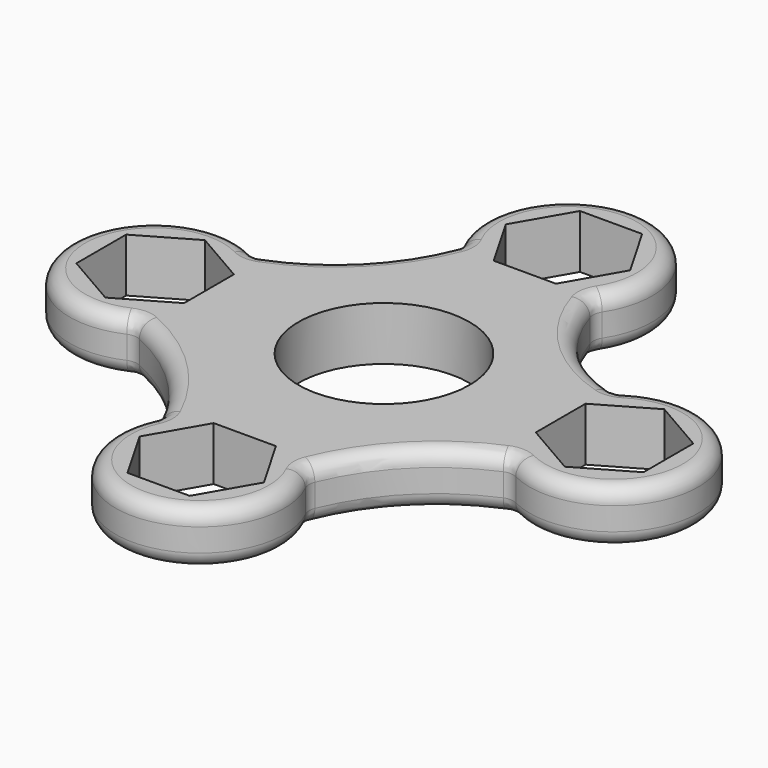
from build123d import *

# Parameters (mm, degrees)
F0_R     = 11.15
F1_DEPTH = 7
F2_F1_R  = 2
F2_F2_R  = 2


with BuildPart() as f1:
    # F0 (on Top) → F1 (new body)
    with BuildSketch(Plane.XY):
        with BuildLine():
            ThreePointArc((23.3964503772, 8.797336664), (14.0846149988, 14.053375372), (8.7316436817, 23.3098282073))
            ThreePointArc((8.7316436817, 23.3098282073), (0.5437011827, 40.9865549206), (-9.3495266884, 24.2046267848))
            ThreePointArc((-9.3495266884, 24.2046267848), (-15.072406885, 15.069278283), (-24.2129318757, 9.3546695572))
            ThreePointArc((-24.2129318757, 9.3546695572), (-40.995618633, 0.310436593), (-24.7499456016, -9.6662779194))
            ThreePointArc((-24.7499456016, -9.6662779194), (-15.7123412284, -15.6876267313), (-9.6305294082, -24.6846539794))
            ThreePointArc((-9.6305294082, -24.6846539794), (0.1339060787, -40.9991849317), (9.4982743355, -24.4517764422))
            ThreePointArc((9.4982743355, -24.4517764422), (15.2376463276, -15.298425789), (24.29093254, -9.4024756707))
            ThreePointArc((24.29093254, -9.4024756707), (40.9867386931, 0.5399748969), (23.3964503772, 8.797336664))
        make_face()
        Polygon((-3.9538544588, -36.8794909641), (-8.0114721507, -29.8514909641), (-3.9538544588, -22.8234909641), (4.1613809249, -22.8234909641), (8.2189986168, -29.8514909641), (4.1613809249, -36.8794909641), align=None, mode=Mode.SUBTRACT)
        Polygon((-36.9018638655, 4.0799905933), (-29.8738638655, 8.1376082852), (-22.8458638655, 4.0799905933), (-22.8458638655, -4.0352447904), (-29.8738638655, -8.0928624823), (-36.9018638655, -4.0352447904), align=None, mode=Mode.SUBTRACT)
        Circle(F0_R, mode=Mode.SUBTRACT)
        Polygon((8.1152353837, 30), (4.0576176919, 22.972), (-4.0576176919, 22.972), (-8.1152353837, 30), (-4.0576176919, 37.028), (4.0576176919, 37.028), align=None, mode=Mode.SUBTRACT)
        Polygon((37.0056270986, -3.9314815574), (29.9776270986, -7.9890992492), (22.9496270986, -3.9314815574), (22.9496270986, 4.1837538264), (29.9776270986, 8.2413715182), (37.0056270986, 4.1837538264), align=None, mode=Mode.SUBTRACT)
    extrude(amount=F1_DEPTH)

    # F2: fillet of radius 2 on 16 edges, made by hand

    # F2_f1
    f2_f1_edges = [f1.edges().sort_by_distance(p)[0] for p in [
        (-24.2129318757, 9.3546695572, 3.5),
        (-24.7499456016, -9.6662779194, 3.5),
        (-9.6305294082, -24.6846539794, 3.5),
        (9.4982743355, -24.4517764422, 3.5),
        (24.29093254, -9.4024756707, 3.5),
        (23.3964503772, 8.797336664, 3.5),
        (8.7316436817, 23.3098282073, 3.5),
        (-9.3495266884, 24.2046267848, 3.5),
    ]]
    fillet(f2_f1_edges, radius=F2_F1_R)

    # F2_f2
    f2_f2_edges = [f1.edges().sort_by_distance(p)[0] for p in [
        (-40.9955957258, 0.3112469049, 0),
        (-40.9955957258, 0.3112469049, 7),
        (0.1503959433, -40.9989718183, 0),
        (0.1503959433, -40.9989718183, 7),
        (40.9864656628, 0.5455018243, 0),
        (40.9864656628, 0.5455018243, 7),
        (0.5287777636, 40.9872832892, 0),
        (0.5287777636, 40.9872832892, 7),
        (8.9372319272, 23.2108101406, 7),
        (-9.5492322972, 24.1305922026, 7),
        (8.9372319272, 23.2108101406, 0),
        (-9.5492322972, 24.1305922026, 0),
        (24.2197549304, -9.6120251278, 7),
        (23.3005316773, 8.992763458, 7),
        (24.2197549304, -9.6120251278, 0),
        (23.3005316773, 8.992763458, 0),
        (-9.8407397297, -24.6243388622, 7),
        (9.6908582331, -24.3838666778, 7),
        (-9.8407397297, -24.6243388622, 0),
        (9.6908582331, -24.3838666778, 0),
        (-24.1390855662, 9.5534890146, 7),
        (-24.6906295336, -9.8697227578, 7),
        (-24.1390855662, 9.5534890146, 0),
        (-24.6906295336, -9.8697227578, 0),
    ]]
    fillet(f2_f2_edges, radius=F2_F2_R)


solid = f1.part
